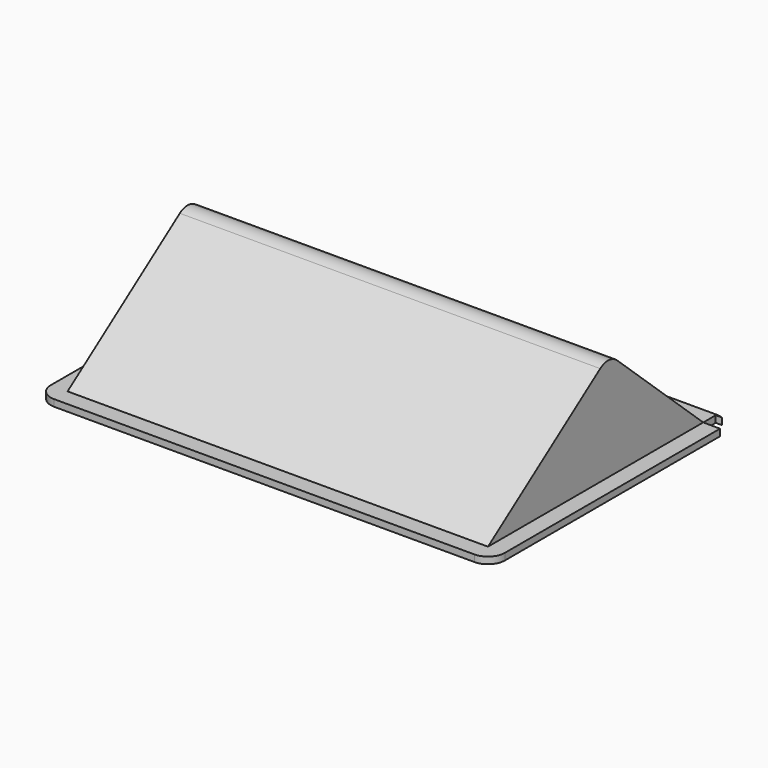
from build123d import *

# Parameters (mm, degrees)
F1_DEPTH    = 79.375
F2_T        = -1.27
F3_W        = 156.21
F3_H        = 97.5264204863
F4_DEPTH    = 2.54
F5_T1_DEPTH = 156.21
F6_W        = 27.2243830562
F6_H        = 5.9061057907
F7_DEPTH    = 25.4


# Not quite as in the source:
# - a fillet or chamfer that OpenCascade refuses, or shapes differently, is made with other operations: its cross-section is extruded or revolved along the edge and cut away or added


with BuildPart() as f1:
    # F0 (on Right) → F1 (new body, symmetric)
    with BuildSketch(Plane.YZ):
        with BuildLine():
            Line((4.3050818061, 37.6678072835), (-48.6652721863, 0))
            Line((-48.6652721863, 0), (52.9347278137, 0))
            Line((52.9347278137, 0), (12.2698422666, 37.1793239287))
            ThreePointArc((12.2698422666, 37.1793239287), (8.3737766286, 38.8309319872), (4.3050818061, 37.6678072835))
        make_face()
    extrude(amount=F1_DEPTH, both=True)

    # F2
    f2_openings = [f1.faces().sort_by_distance(p)[0] for p in [
        (0, 2.134728, 0),
    ]]
    offset(amount=F2_T, openings=f2_openings)

    # F3 (on face) → F4 (join)
    with BuildSketch(Plane(origin=(0, 0, 0), x_dir=(1, 0, 0), z_dir=(0, 0, -1))):
        with BuildLine():
            Line((79.375, 55.0152721863), (-79.375, 55.0152721863))
            ThreePointArc((-79.375, 55.0152721863), (-83.8651280605, 53.1554002469), (-85.725, 48.6652721863))
            Line((-85.725, 48.6652721863), (-85.725, -52.9347278137))
            ThreePointArc((-85.725, -52.9347278137), (-83.8651280605, -57.4248558742), (-79.375, -59.2847278137))
            Line((-79.375, -59.2847278137), (79.375, -59.2847278137))
            ThreePointArc((79.375, -59.2847278137), (83.8651280605, -57.4248558742), (85.725, -52.9347278137))
            Line((85.725, -52.9347278137), (85.725, 48.6652721863))
            ThreePointArc((85.725, 48.6652721863), (83.8651280605, 53.1554002469), (79.375, 55.0152721863))
        make_face()
        with Locations((0, -2.2893925404)):
            Rectangle(F3_W, F3_H, mode=Mode.SUBTRACT)
    extrude(amount=F4_DEPTH)

    # F5: fillet of radius 7.62 on 2 edges, made by hand

    # F5_s2 → F5_t1 (cut)
    with BuildSketch(Plane.YZ.offset(-78.105)):
        with BuildLine():
            ThreePointArc((-52.1538622168, -2.5404), (-49.042649841, -1.8764456481), (-46.4735195754, -0.0002666836))
            Line((-46.4735195754, -0.0002666836), (-45.9054853113, -0.5083899205))
            ThreePointArc((-45.9054853113, -0.5083899205), (-45.7116811342, -1.2701333418), (-45.7116811342, -2.54))
            Line((-45.7116811342, -2.54), (-46.4738177027, -3.3021365685))
            ThreePointArc((-46.4738177027, -3.3021365685), (-49.3138399597, -3.3021365685), (-52.1538622168, -3.3025365685))
            Line((-52.1538622168, -3.3025365685), (-52.1538622168, -2.5404))
        make_face()
        with BuildLine():
            ThreePointArc((56.7326472976, -2.5404), (53.6214349219, -1.8764456481), (51.0523046563, -0.0002666836))
            Line((51.0523046563, -0.0002666836), (50.4842703921, -0.5083899205))
            ThreePointArc((50.4842703921, -0.5083899205), (50.290466215, -1.2701333418), (50.290466215, -2.54))
            Line((50.290466215, -2.54), (51.0526027836, -3.3021365685))
            ThreePointArc((51.0526027836, -3.3021365685), (53.8926250406, -3.3021365685), (56.7326472976, -3.3025365685))
            Line((56.7326472976, -3.3025365685), (56.7326472976, -2.5404))
        make_face()
    extrude(amount=F5_T1_DEPTH, mode=Mode.SUBTRACT)

    # F6 (on face) → F7 (cut)
    with BuildSketch(Plane(origin=(0, 0, -2.54), x_dir=(1, 0, 0), z_dir=(0, 0, -1))):
        with Locations((92.9871915281, -55.887780709)):
            Rectangle(F6_W, F6_H)
    extrude(amount=-F7_DEPTH, mode=Mode.SUBTRACT)


solid = f1.part
